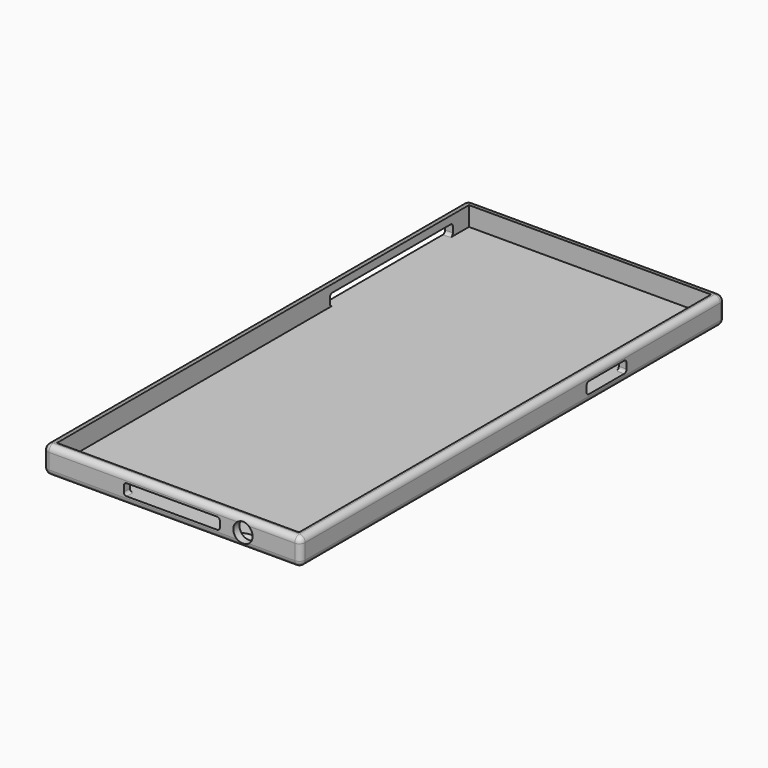
from build123d import *

# Parameters (mm, degrees)
F0_W          = 67
F0_H          = 138
F1_DEPTH      = 7
F2_T          = -2
F4_DEPTH      = 2
F6_DEPTH      = 2
F8_DEPTH      = 2
F10_D         = 5
F10_DEPTH     = 2
F10_TIP       = 1.5021515476
F11_T1_DEPTH  = 135
F11_T3_DEPTH  = 64
F11_T5_DEPTH  = 4
F11_S9_W      = 1.5
F11_S9_H      = 1.5
F11_T10_DEPTH = 1.5
F11_S15_W     = 1.5
F11_S15_H     = 1.5
F11_T16_DEPTH = 1.5
F11_S21_W     = 1.5
F11_S21_H     = 1.5
F11_T22_DEPTH = 1.5
F11_S27_W     = 1.5
F11_S27_H     = 1.5
F11_T28_DEPTH = 1.5
F11_S33_W     = 1.5
F11_S33_H     = 1.5
F11_T34_DEPTH = 1.5
F11_S39_W     = 1.5
F11_S39_H     = 1.5
F11_T40_DEPTH = 1.5
F11_S45_W     = 1.5
F11_S45_H     = 1.5
F11_T46_DEPTH = 1.5
F11_S51_W     = 1.5
F11_S51_H     = 1.5
F11_T52_DEPTH = 1.5


# Not quite as in the source:
# - a fillet or chamfer that OpenCascade refuses, or shapes differently, is made with other operations: its cross-section is extruded or revolved along the edge and cut away or added


with BuildPart() as f1:
    # F0 (on Top) → F1 (new body)
    with BuildSketch(Plane.XY):
        Rectangle(F0_W, F0_H)
    extrude(amount=F1_DEPTH)

    # F2
    f2_openings = [f1.faces().sort_by_distance(p)[0] for p in [
        (0, 0, 7),
    ]]
    offset(amount=F2_T, openings=f2_openings)

    # F3 (on face) → F4 (cut, through all)
    with BuildSketch(Plane(origin=(-33.5, 0, 0), x_dir=(0, -1, 0), z_dir=(-1, 0, 0))):
        with BuildLine():
            Line((-22.538946541, 5), (-61.0191351455, 5))
            ThreePointArc((-61.0191351455, 5), (-61.5564696174, 4.7774287742), (-61.7790408432, 4.2400943022))
            Line((-61.7790408432, 4.2400943022), (-61.7790408432, 2.7599056978))
            ThreePointArc((-61.7790408432, 2.7599056978), (-61.5564696174, 2.2225712258), (-61.0191351455, 2))
            Line((-61.0191351455, 2), (-22.538946541, 2))
            ThreePointArc((-22.538946541, 2), (-22.0016120691, 2.2225712258), (-21.7790408432, 2.7599056978))
            Line((-21.7790408432, 2.7599056978), (-21.7790408432, 4.2400943022))
            ThreePointArc((-21.7790408432, 4.2400943022), (-22.0016120691, 4.7774287742), (-22.538946541, 5))
        make_face()
    extrude(amount=-F4_DEPTH, mode=Mode.SUBTRACT)

    # F5 (on face) → F6 (cut, through all)
    with BuildSketch(Plane.YZ.offset(33.5)):
        with BuildLine():
            Line((36.2400943022, 5), (24.7599056978, 5))
            ThreePointArc((24.7599056978, 5), (24.2225712258, 4.7774287742), (24, 4.2400943022))
            Line((24, 4.2400943022), (24, 2.7599056978))
            ThreePointArc((24, 2.7599056978), (24.2225712258, 2.2225712258), (24.7599056978, 2))
            Line((24.7599056978, 2), (36.2400943022, 2))
            ThreePointArc((36.2400943022, 2), (36.7774287742, 2.2225712258), (37, 2.7599056978))
            Line((37, 2.7599056978), (37, 4.2400943022))
            ThreePointArc((37, 4.2400943022), (36.7774287742, 4.7774287742), (36.2400943022, 5))
        make_face()
    extrude(amount=-F6_DEPTH, mode=Mode.SUBTRACT)

    # F7 (on face) → F8 (cut, through all)
    with BuildSketch(Plane.XZ.offset(69)):
        with BuildLine():
            Line((11.7400943022, 5), (-11.7400943022, 5))
            ThreePointArc((-11.7400943022, 5), (-12.2774287742, 4.7774287742), (-12.5, 4.2400943022))
            Line((-12.5, 4.2400943022), (-12.5, 2.7599056978))
            ThreePointArc((-12.5, 2.7599056978), (-12.2774287742, 2.2225712258), (-11.7400943022, 2))
            Line((-11.7400943022, 2), (11.7400943022, 2))
            ThreePointArc((11.7400943022, 2), (12.2774287742, 2.2225712258), (12.5, 2.7599056978))
            Line((12.5, 2.7599056978), (12.5, 4.2400943022))
            ThreePointArc((12.5, 4.2400943022), (12.2774287742, 4.7774287742), (11.7400943022, 5))
        make_face()
    extrude(amount=-F8_DEPTH, mode=Mode.SUBTRACT)

    # F10
    with Locations(Plane.XZ.offset(69)):
        with Locations((18.5, 3.5)):
            Hole(F10_D / 2, depth=F10_DEPTH)
            with Locations((0, 0, -(F10_DEPTH + F10_TIP / 2))):  # 118° drill point
                Cone(0, F10_D / 2, F10_TIP, mode=Mode.SUBTRACT)

    # F11: fillet of radius 1.5 on 12 edges, made by hand

    # F11_s2 → F11_t1 (cut)
    with BuildSketch(Plane.XZ.offset(-67.5)):
        with BuildLine():
            ThreePointArc((33.5, 5.5), (33.0606601718, 6.5606601718), (32, 7))
            Line((32, 7), (33.5, 7))
            Line((33.5, 7), (33.5, 5.5))
        make_face()
        with BuildLine():
            ThreePointArc((33.5, 1.5), (33.0606601718, 0.4393398282), (32, 0))
            Line((32, 0), (33.5, 0))
            Line((33.5, 0), (33.5, 1.5))
        make_face()
        with BuildLine():
            ThreePointArc((-32, 7), (-33.0606601718, 6.5606601718), (-33.5, 5.5))
            Line((-33.5, 5.5), (-33.5, 7))
            Line((-33.5, 7), (-32, 7))
        make_face()
        with BuildLine():
            ThreePointArc((-32, 0), (-33.0606601718, 0.4393398282), (-33.5, 1.5))
            Line((-33.5, 1.5), (-33.5, 0))
            Line((-33.5, 0), (-32, 0))
        make_face()
    extrude(amount=F11_T1_DEPTH, mode=Mode.SUBTRACT)

    # F11_s4 → F11_t3 (cut)
    with BuildSketch(Plane.YZ.offset(-32)):
        with BuildLine():
            ThreePointArc((-69, 5.5), (-68.5606601718, 6.5606601718), (-67.5, 7))
            Line((-67.5, 7), (-69, 7))
            Line((-69, 7), (-69, 5.5))
        make_face()
        with BuildLine():
            ThreePointArc((-69, 1.5), (-68.5606601718, 0.4393398282), (-67.5, 0))
            Line((-67.5, 0), (-69, 0))
            Line((-69, 0), (-69, 1.5))
        make_face()
        with BuildLine():
            ThreePointArc((67.5, 7), (68.5606601718, 6.5606601718), (69, 5.5))
            Line((69, 5.5), (69, 7))
            Line((69, 7), (67.5, 7))
        make_face()
        with BuildLine():
            ThreePointArc((67.5, 0), (68.5606601718, 0.4393398282), (69, 1.5))
            Line((69, 1.5), (69, 0))
            Line((69, 0), (67.5, 0))
        make_face()
    extrude(amount=F11_T3_DEPTH, mode=Mode.SUBTRACT)

    # F11_s6 → F11_t5 (cut)
    with BuildSketch(Plane.XY.offset(1.5)):
        with BuildLine():
            ThreePointArc((33.5, -67.5), (33.0606601718, -68.5606601718), (32, -69))
            Line((32, -69), (33.5, -69))
            Line((33.5, -69), (33.5, -67.5))
        make_face()
        with BuildLine():
            ThreePointArc((33.5, 67.5), (33.0606601718, 68.5606601718), (32, 69))
            Line((32, 69), (33.5, 69))
            Line((33.5, 69), (33.5, 67.5))
        make_face()
        with BuildLine():
            ThreePointArc((-32, 69), (-33.0606601718, 68.5606601718), (-33.5, 67.5))
            Line((-33.5, 67.5), (-33.5, 69))
            Line((-33.5, 69), (-32, 69))
        make_face()
        with BuildLine():
            ThreePointArc((-32, -69), (-33.0606601718, -68.5606601718), (-33.5, -67.5))
            Line((-33.5, -67.5), (-33.5, -69))
            Line((-33.5, -69), (-32, -69))
        make_face()
    extrude(amount=F11_T5_DEPTH, mode=Mode.SUBTRACT)


with BuildPart() as f11_tool8:
    # F11_s9 → F11_t10 (new body)
    with BuildSketch(Plane.YZ.offset(32)):
        with Locations((-68.25, 6.25)):
            Rectangle(F11_S9_W, F11_S9_H)
    extrude(amount=F11_T10_DEPTH)

    # F11_s11 → F11_t12 (revolve, cut)
    with BuildSketch(Plane(origin=(32, -67.5, 5.5), x_dir=(0, 0.7071067812, -0.7071067812), z_dir=(0, -0.7071067812, -0.7071067812))):
        with BuildLine():
            ThreePointArc((0, -1.5), (1.5, 0), (0, 1.5))
            Line((0, 1.5), (0, -1.5))
        make_face()
    revolve(axis=Axis((32, -67.5, 5.5), (1, 0, 0)), mode=Mode.SUBTRACT)


with BuildPart() as f1_1:
    add(f1.part)

    # F11_t7: cut F11_tool8
    add(f11_tool8.part, mode=Mode.SUBTRACT)


with BuildPart() as f11_tool14:
    # F11_s15 → F11_t16 (new body)
    with BuildSketch(Plane.YZ.offset(32)):
        with Locations((68.25, 6.25)):
            Rectangle(F11_S15_W, F11_S15_H)
    extrude(amount=F11_T16_DEPTH)

    # F11_s17 → F11_t18 (revolve, cut)
    with BuildSketch(Plane(origin=(32, 67.5, 5.5), x_dir=(0, -0.7071067812, -0.7071067812), z_dir=(0, -0.7071067812, 0.7071067812))):
        with BuildLine():
            ThreePointArc((0, -1.5), (1.5, 0), (0, 1.5))
            Line((0, 1.5), (0, -1.5))
        make_face()
    revolve(axis=Axis((32, 67.5, 5.5), (1, 0, 0)), mode=Mode.SUBTRACT)


with BuildPart() as f1_2:
    add(f1_1.part)

    # F11_t13: cut F11_tool14
    add(f11_tool14.part, mode=Mode.SUBTRACT)


with BuildPart() as f11_tool20:
    # F11_s21 → F11_t22 (new body)
    with BuildSketch(Plane.XZ.offset(67.5)):
        with Locations((-32.75, 6.25)):
            Rectangle(F11_S21_W, F11_S21_H)
    extrude(amount=F11_T22_DEPTH)

    # F11_s23 → F11_t24 (revolve, cut)
    with BuildSketch(Plane(origin=(-32, -67.5, 5.5), x_dir=(0.7071067812, 0, -0.7071067812), z_dir=(-0.7071067812, 0, -0.7071067812))):
        with BuildLine():
            ThreePointArc((0, -1.5), (1.5, 0), (0, 1.5))
            Line((0, 1.5), (0, -1.5))
        make_face()
    revolve(axis=Axis((-32, -67.5, 5.5), (0, -1, 0)), mode=Mode.SUBTRACT)


with BuildPart() as f1_3:
    add(f1_2.part)

    # F11_t19: cut F11_tool20
    add(f11_tool20.part, mode=Mode.SUBTRACT)


with BuildPart() as f11_tool26:
    # F11_s27 → F11_t28 (new body)
    with BuildSketch(Plane.XZ.offset(67.5)):
        with Locations((-32.75, 0.75)):
            Rectangle(F11_S27_W, F11_S27_H)
    extrude(amount=F11_T28_DEPTH)

    # F11_s29 → F11_t30 (revolve, cut)
    with BuildSketch(Plane(origin=(-32, -67.5, 1.5), x_dir=(0.7071067812, 0, 0.7071067812), z_dir=(0.7071067812, 0, -0.7071067812))):
        with BuildLine():
            ThreePointArc((0, -1.5), (1.5, 0), (0, 1.5))
            Line((0, 1.5), (0, -1.5))
        make_face()
    revolve(axis=Axis((-32, -67.5, 1.5), (0, -1, 0)), mode=Mode.SUBTRACT)


with BuildPart() as f1_4:
    add(f1_3.part)

    # F11_t25: cut F11_tool26
    add(f11_tool26.part, mode=Mode.SUBTRACT)


with BuildPart() as f11_tool32:
    # F11_s33 → F11_t34 (new body)
    with BuildSketch(Plane.YZ.offset(32)):
        with Locations((-68.25, 0.75)):
            Rectangle(F11_S33_W, F11_S33_H)
    extrude(amount=F11_T34_DEPTH)

    # F11_s35 → F11_t36 (revolve, cut)
    with BuildSketch(Plane(origin=(32, -67.5, 1.5), x_dir=(0, 0.7071067812, 0.7071067812), z_dir=(0, 0.7071067812, -0.7071067812))):
        with BuildLine():
            ThreePointArc((0, -1.5), (1.5, 0), (0, 1.5))
            Line((0, 1.5), (0, -1.5))
        make_face()
    revolve(axis=Axis((32, -67.5, 1.5), (1, 0, 0)), mode=Mode.SUBTRACT)


with BuildPart() as f1_5:
    add(f1_4.part)

    # F11_t31: cut F11_tool32
    add(f11_tool32.part, mode=Mode.SUBTRACT)


with BuildPart() as f11_tool38:
    # F11_s39 → F11_t40 (new body)
    with BuildSketch(Plane.YZ.offset(32)):
        with Locations((68.25, 0.75)):
            Rectangle(F11_S39_W, F11_S39_H)
    extrude(amount=F11_T40_DEPTH)

    # F11_s41 → F11_t42 (revolve, cut)
    with BuildSketch(Plane(origin=(32, 67.5, 1.5), x_dir=(0, -0.7071067812, 0.7071067812), z_dir=(0, 0.7071067812, 0.7071067812))):
        with BuildLine():
            ThreePointArc((0, -1.5), (1.5, 0), (0, 1.5))
            Line((0, 1.5), (0, -1.5))
        make_face()
    revolve(axis=Axis((32, 67.5, 1.5), (1, 0, 0)), mode=Mode.SUBTRACT)


with BuildPart() as f1_6:
    add(f1_5.part)

    # F11_t37: cut F11_tool38
    add(f11_tool38.part, mode=Mode.SUBTRACT)


with BuildPart() as f11_tool44:
    # F11_s45 → F11_t46 (new body)
    with BuildSketch(Plane.XY.offset(5.5)):
        with Locations((-32.75, 68.25)):
            Rectangle(F11_S45_W, F11_S45_H)
    extrude(amount=F11_T46_DEPTH)

    # F11_s47 → F11_t48 (revolve, cut)
    with BuildSketch(Plane(origin=(-32, 67.5, 5.5), x_dir=(0.7071067812, -0.7071067812, 0), z_dir=(-0.7071067812, -0.7071067812, 0))):
        with BuildLine():
            ThreePointArc((0, -1.5), (1.5, 0), (0, 1.5))
            Line((0, 1.5), (0, -1.5))
        make_face()
    revolve(axis=Axis((-32, 67.5, 5.5), (0, 0, 1)), mode=Mode.SUBTRACT)


with BuildPart() as f1_7:
    add(f1_6.part)

    # F11_t43: cut F11_tool44
    add(f11_tool44.part, mode=Mode.SUBTRACT)


with BuildPart() as f11_tool50:
    # F11_s51 → F11_t52 (new body)
    with BuildSketch(Plane.XY.offset(1.5)):
        with Locations((-32.75, 68.25)):
            Rectangle(F11_S51_W, F11_S51_H)
    extrude(amount=-F11_T52_DEPTH)

    # F11_s53 → F11_t54 (revolve, cut)
    with BuildSketch(Plane(origin=(-32, 67.5, 1.5), x_dir=(0.7071067812, -0.7071067812, 0), z_dir=(0.7071067812, 0.7071067812, 0))):
        with BuildLine():
            ThreePointArc((0, -1.5), (1.5, 0), (0, 1.5))
            Line((0, 1.5), (0, -1.5))
        make_face()
    revolve(axis=Axis((-32, 67.5, 1.5), (0, 0, -1)), mode=Mode.SUBTRACT)


with BuildPart() as f1_8:
    add(f1_7.part)

    # F11_t49: cut F11_tool50
    add(f11_tool50.part, mode=Mode.SUBTRACT)


solid = f1_8.part
